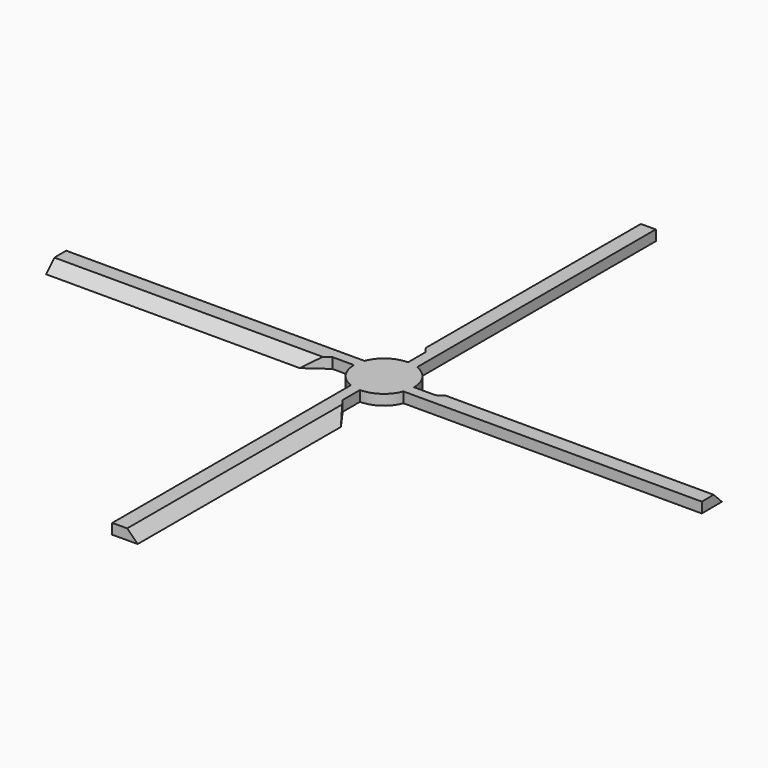
from build123d import *

# Parameters (mm, degrees)
F1_DEPTH = 1.016
F2_SIZE  = 1.01599


# Not quite as in the source:
# - a fillet or chamfer is up to 0.001 mm smaller than in the source, because OpenCascade refuses the exact size


with BuildPart() as f1:
    # F0 (on Top) → F1 (new body)
    with BuildSketch(Plane.XY):
        with BuildLine():
            ThreePointArc((0, 2.9195159057), (0.527538065, 2.8714589869), (1.0377089673, 2.7288703199))
            Line((1.0377089673, 2.7288703199), (1.0377089673, 31.7330373601))
            Line((1.0377089673, 31.7330373601), (-1.4246536514, 31.7180210917))
            Line((-1.4246536514, 31.7180210917), (-1.4426441077, 7.0411415527))
            Line((-1.4426441077, 7.0411415527), (0, 5.0220009871))
            Line((0, 5.0220009871), (0, 2.9195159057))
        make_face()
        with BuildLine():
            Line((1.0377089673, 1.7452047762), (1.0377089673, 2.7288703199))
            ThreePointArc((1.0377089673, 2.7288703199), (0.527538065, 2.8714589869), (0, 2.9195159057))
            Line((0, 2.9195159057), (1.0377089673, 1.7452047762))
        make_face()
        with BuildLine():
            Line((1.7452047762, -1.0377089673), (2.9195159057, 0))
            ThreePointArc((2.9195159057, 0), (2.4034538646, 1.6574023784), (1.0377089673, 2.7288703199))
            Line((1.0377089673, 2.7288703199), (1.0377089673, 1.7452047762))
            Line((1.0377089673, 1.7452047762), (0, 2.9195159057))
            ThreePointArc((0, 2.9195159057), (-1.6574023784, 2.4034538646), (-2.7288703199, 1.0377089673))
            Line((-2.7288703199, 1.0377089673), (-1.7452047762, 1.0377089673))
            Line((-1.7452047762, 1.0377089673), (-2.9195159057, 0))
            ThreePointArc((-2.9195159057, 0), (-2.4034538646, -1.6574023784), (-1.0377089673, -2.7288703199))
            Line((-1.0377089673, -2.7288703199), (-1.0377089673, -1.7452047762))
            Line((-1.0377089673, -1.7452047762), (0, -2.9195159057))
            ThreePointArc((0, -2.9195159057), (1.6574023784, -2.4034538646), (2.7288703199, -1.0377089673))
            Line((2.7288703199, -1.0377089673), (1.7452047762, -1.0377089673))
        make_face()
        with BuildLine():
            Line((-1.7452047762, 1.0377089673), (-2.7288703199, 1.0377089673))
            ThreePointArc((-2.7288703199, 1.0377089673), (-2.8714589869, 0.527538065), (-2.9195159057, 0))
            Line((-2.9195159057, 0), (-1.7452047762, 1.0377089673))
        make_face()
        with BuildLine():
            ThreePointArc((2.7288703199, -1.0377089673), (2.8714589869, -0.527538065), (2.9195159057, 0))
            Line((2.9195159057, 0), (1.7452047762, -1.0377089673))
            Line((1.7452047762, -1.0377089673), (2.7288703199, -1.0377089673))
        make_face()
        with BuildLine():
            Line((5.0220009871, 0), (2.9195159057, 0))
            ThreePointArc((2.9195159057, 0), (2.8714589869, -0.527538065), (2.7288703199, -1.0377089673))
            Line((2.7288703199, -1.0377089673), (31.7330373601, -1.0377089673))
            Line((31.7330373601, -1.0377089673), (31.7180210917, 1.4246536514))
            Line((31.7180210917, 1.4246536514), (7.0411415527, 1.4426441077))
            Line((7.0411415527, 1.4426441077), (5.0220009871, 0))
        make_face()
        with BuildLine():
            ThreePointArc((-1.0377089673, -2.7288703199), (-0.527538065, -2.8714589869), (0, -2.9195159057))
            Line((0, -2.9195159057), (-1.0377089673, -1.7452047762))
            Line((-1.0377089673, -1.7452047762), (-1.0377089673, -2.7288703199))
        make_face()
        with BuildLine():
            Line((0, -5.0220009871), (0, -2.9195159057))
            ThreePointArc((0, -2.9195159057), (-0.527538065, -2.8714589869), (-1.0377089673, -2.7288703199))
            Line((-1.0377089673, -2.7288703199), (-1.0377089673, -31.7330373601))
            Line((-1.0377089673, -31.7330373601), (1.4246536514, -31.7180210917))
            Line((1.4246536514, -31.7180210917), (1.4426441077, -7.0411415527))
            Line((1.4426441077, -7.0411415527), (0, -5.0220009871))
        make_face()
        with BuildLine():
            ThreePointArc((-2.9195159057, 0), (-2.8714589869, 0.527538065), (-2.7288703199, 1.0377089673))
            Line((-2.7288703199, 1.0377089673), (-31.7330373601, 1.0377089673))
            Line((-31.7330373601, 1.0377089673), (-31.7180210917, -1.4246536514))
            Line((-31.7180210917, -1.4246536514), (-7.0411415527, -1.4426441077))
            Line((-7.0411415527, -1.4426441077), (-5.0220009871, 0))
            Line((-5.0220009871, 0), (-2.9195159057, 0))
        make_face()
    extrude(amount=F1_DEPTH)

    # F2 (size 1.016 in the source; OpenCascade refuses exactly that, so slightly less here)
    f2_edges = [f1.edges().sort_by_distance(p)[0] for p in [
        (-19.379581, -1.433649, 1.016),
        (1.433649, -19.379581, 1.016),
        (19.379581, 1.433649, 1.016),
        (-1.433649, 19.379581, 1.016),
    ]]
    chamfer(f2_edges, length=F2_SIZE)


solid = f1.part
